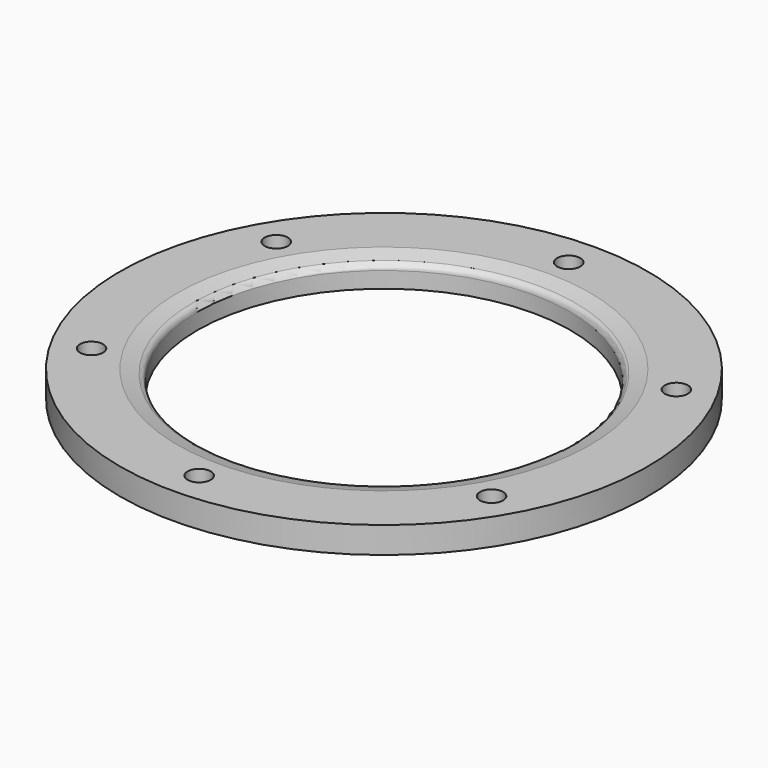
from build123d import *

# Parameters (mm, degrees)
F2_R            = 7
F3_DEPTH        = 25
F3_COPIES_COUNT = 6


# Not quite as in the source:
# - a pattern or mirror of a feature is missing from the dataset's text; its kind, count and spacing are read off the source's solid


with BuildPart() as f1:
    # F0 (on Right) → F1 (revolve)
    with BuildSketch(Plane.YZ):
        with BuildLine():
            Line((160, 16), (125, 16))
            Line((125, 16), (115.9647238196, 13.5790050441))
            ThreePointArc((115.9647238196, 13.5790050441), (113.8265866388, 12.1503474549), (113, 9.7153017389))
            Line((113, 9.7153017389), (113, 0))
            Line((113, 0), (160, 0))
            Line((160, 0), (160, 16))
        make_face()
    revolve(axis=Axis((0, 0, -1.8696532477), (0, 0, -1)))

    # F2 (on face) → F3 (cut)
    with BuildSketch(Plane.XY.offset(16)):
        with Locations((0, 140)):
            Circle(F2_R)
    f3 = extrude(amount=-F3_DEPTH, mode=Mode.SUBTRACT)

    # F3_copies: F3 ×6 about axis
    f3_copies_axis = Axis((0, 0, 0), (0, 0, 1))
    for i in range(1, F3_COPIES_COUNT):
        add(f3.rotate(f3_copies_axis, i * 360 / F3_COPIES_COUNT), mode=Mode.SUBTRACT)


solid = f1.part
